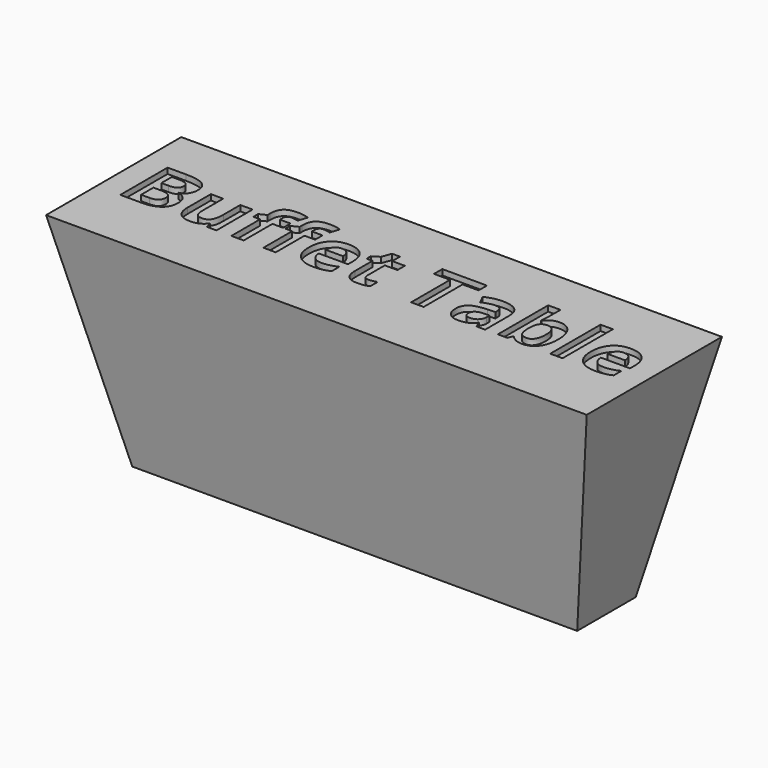
from build123d import *

# Parameters (mm, degrees)
F0_W         = 2438.4
F0_H         = 762
F1_DEPTH     = 1016
F1_TAPER     = 12
F2_TEXT_SIZE = 373.415007657
F3_DEPTH     = 25.4


# Not quite as in the source:
# - Text() gives the source's letters only with a copy of the font that has no kerning and outlines rounded to 1/6400 em; it was checked with that copy


with BuildPart() as f1:
    # F0 (on Top) → F1 (new body)
    with BuildSketch(Plane.XY):
        Rectangle(F0_W, F0_H)
    extrude(amount=-F1_DEPTH, taper=F1_TAPER)

    # F2 (on face) → F3 (cut)
    with BuildSketch(Plane.XY):
        with Locations((-1144.9535126378, -97.3458011148)):
            Text('Buffet Table', F2_TEXT_SIZE, font='Open Sans', font_style=FontStyle.BOLD, text_align=(TextAlign.LEFT, TextAlign.BOTTOM))
    extrude(amount=-F3_DEPTH, mode=Mode.SUBTRACT)


solid = f1.part
